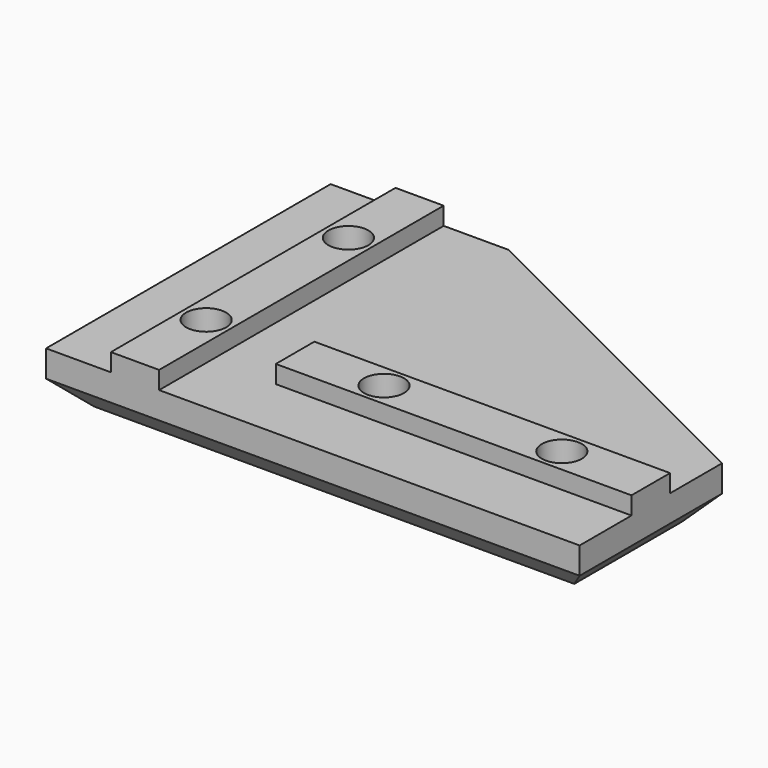
from build123d import *

# Parameters (mm, degrees)
F1_DEPTH = 6
F3_DEPTH = 2
F4_R     = 2.25
F5_DEPTH = 8.001
F6_R     = 3.75
F7_DEPTH = 2
F8_SIZE  = 3


with BuildPart() as f1:
    # F0 (on Top) → F1 (new body)
    with BuildSketch(Plane.XY):
        Polygon((0, 40), (0, 0), (60, 0), (60, 20), (20, 40), align=None)
    extrude(amount=F1_DEPTH)

    # F2 (on face) → F3 (join)
    with BuildSketch(Plane.XY.offset(6)):
        Polygon((12.71, 40), (7.29, 40), (7.29, 0), (10, 0), (12.71, 0), align=None)
        Polygon((60, 7.29), (60, 12.71), (20, 12.71), (20, 10), (20, 7.29), align=None)
    extrude(amount=F3_DEPTH)

    # F4 (on face) → F5 (cut, through all)
    with BuildSketch(Plane(origin=(0, 0, 0), x_dir=(1, 0, 0), z_dir=(0, 0, -1))):
        with Locations((10, -10)):
            Circle(F4_R)
        with Locations((50, -10)):
            Circle(F4_R)
        with Locations((10, -30)):
            Circle(F4_R)
        with Locations((30, -10)):
            Circle(F4_R)
    extrude(amount=-F5_DEPTH, mode=Mode.SUBTRACT)

    # F6 (on face) → F7 (cut)
    with BuildSketch(Plane(origin=(0, 0, 0), x_dir=(1, 0, 0), z_dir=(0, 0, -1))):
        with Locations((10, -10)):
            Circle(F6_R)
        with Locations((30, -10)):
            Circle(F6_R)
        with Locations((50, -10)):
            Circle(F6_R)
        with Locations((10, -30)):
            Circle(F6_R)
    extrude(amount=-F7_DEPTH, mode=Mode.SUBTRACT)

    # F8
    f8_edges = [f1.edges().sort_by_distance(p)[0] for p in [
        (30, 0, 0),
        (0, 20, 0),
        (60, 10, 0),
        (10, 40, 0),
        (40, 30, 0),
    ]]
    chamfer(f8_edges, length=F8_SIZE)


solid = f1.part
